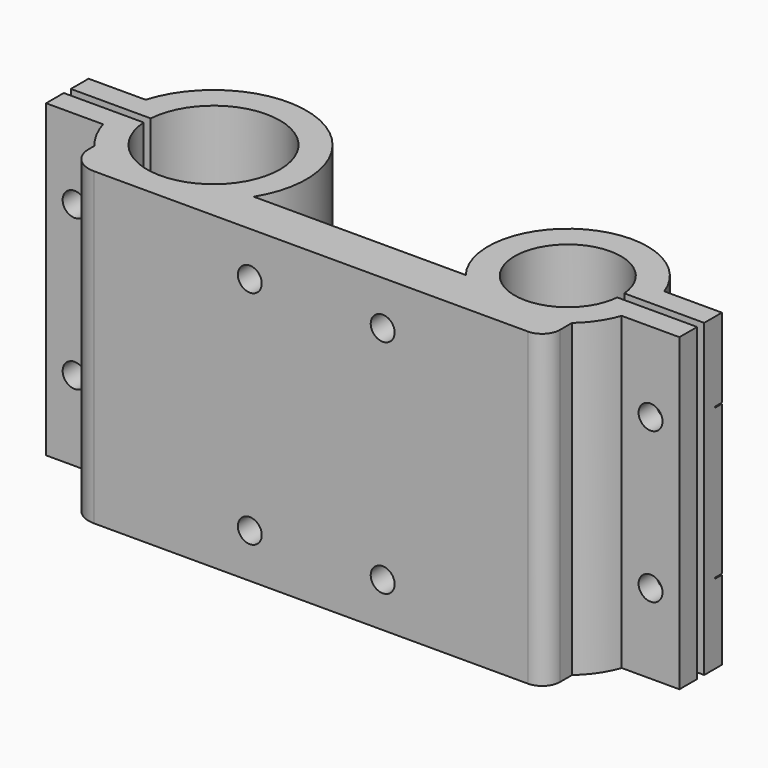
from build123d import *

# Parameters (mm, degrees)
F1_DEPTH   = 35
F3_D       = 2.7
F5_DEPTH   = 1
F6_DEPTH   = 1
F9_D       = 2.7
F9_ON_F7_D = 2.7
F8_W       = 1.6217698948
F8_H       = 2.85
F10_DEPTH  = 1
F11_DEPTH  = 1


# Not quite as in the source:
# - a feature names something its author has since deleted; it is built from what else it names


with BuildPart() as f1:
    # F0 (on Top) → F1 (new body)
    with BuildSketch(Plane.XY):
        with BuildLine():
            Line((-21.3074208284, -25.7097307226), (-27.8221394541, -25.7097307226))
            ThreePointArc((-27.8221394541, -25.7097307226), (-41.1900200037, -21.1492925546), (-42.5323706273, -35.2097307226))
            Line((-42.5323706273, -35.2097307226), (-68.0612095771, -35.2097307226))
            ThreePointArc((-68.0612095771, -35.2097307226), (-71.4714049121, -19.3897012131), (-86.3697267271, -25.7097307226))
            Line((-86.3697267271, -25.7097307226), (-92.8074208284, -25.7097307226))
            Line((-92.8074208284, -25.7097307226), (-92.8074208284, -28.2097307226))
            Line((-92.8074208284, -28.2097307226), (-83.7907356019, -28.2097307226))
            ThreePointArc((-83.7907356019, -28.2097307226), (-68.8074208284, -28.7097307226), (-83.7907356019, -29.2097307226))
            Line((-83.7907356019, -29.2097307226), (-92.8074208284, -29.2097307226))
            Line((-92.8074208284, -29.2097307226), (-92.8074208284, -31.7097307226))
            Line((-92.8074208284, -31.7097307226), (-86.3697267271, -31.7097307226))
            ThreePointArc((-86.3697267271, -31.7097307226), (-85.5676654464, -33.6592629847), (-84.3923404334, -35.4092885424))
            Line((-84.3923404334, -35.4092885424), (-84.3923404334, -36.2097307226))
            ThreePointArc((-84.3923404334, -36.2097307226), (-83.5136607769, -38.3310510662), (-81.3923404334, -39.2097307226))
            Line((-81.3923404334, -39.2097307226), (-32.3990289542, -39.2097307226))
            ThreePointArc((-32.3990289542, -39.2097307226), (-30.9848153918, -38.623944285), (-30.3990289542, -37.2097307226))
            Line((-30.3990289542, -37.2097307226), (-30.3990289542, -35.4987590376))
            ThreePointArc((-30.3990289542, -35.4987590376), (-28.8654021984, -33.7709913079), (-27.8221394541, -31.7097307226))
            Line((-27.8221394541, -31.7097307226), (-21.3074208284, -31.7097307226))
            Line((-21.3074208284, -31.7097307226), (-21.3074208284, -29.2097307226))
            Line((-21.3074208284, -29.2097307226), (-30.3282904568, -29.2097307226))
            ThreePointArc((-30.3282904568, -29.2097307226), (-42.3074208284, -28.7097307226), (-30.3282904568, -28.2097307226))
            Line((-30.3282904568, -28.2097307226), (-21.3074208284, -28.2097307226))
            Line((-21.3074208284, -28.2097307226), (-21.3074208284, -25.7097307226))
        make_face()
    extrude(amount=F1_DEPTH)

    # F3 (through all)
    with Locations(Plane.XZ.offset(39.2097307226)):
        with Locations((-63.8074208284, 30), (-48.80741708, 30), (-48.80741708, 5), (-63.8074208284, 5)):
            Hole(F3_D / 2)

    # F4 (on face) → F5 (cut)
    with BuildSketch(Plane(origin=(0, -35.2097307226, 0), x_dir=(-1, 0, 0), z_dir=(0, 1, 0))):
        Polygon((50.4817328606, 27.1), (52.1560486413, 30), (50.4817328606, 32.9), (47.1331012993, 32.9), (45.4587855187, 30), (47.1331012993, 27.1), align=None)
        Polygon((62.1331050477, 32.9), (60.4587892671, 30), (62.1331050477, 27.1), (65.481736609, 27.1), (67.1560523897, 30), (65.481736609, 32.9), align=None)
        Polygon((52.1560486413, 5), (50.4817328606, 7.9), (47.1331012993, 7.9), (45.4587855187, 5), (47.1331012993, 2.1), (50.4817328606, 2.1), align=None)
        Polygon((62.1331050477, 2.1), (65.481736609, 2.1), (67.1560523897, 5), (65.481736609, 7.9), (62.1331050477, 7.9), (60.4587892671, 5), align=None)
    extrude(amount=-F5_DEPTH, mode=Mode.SUBTRACT)

    # F6 (add): a face of the model
    f6_faces = [f1.faces().sort_by_distance(p)[0] for p in [
        (-55.1452142049, -35.2097307226, 17.5),
    ]]
    extrude(f6_faces, amount=F6_DEPTH)

    # F9 (through all)
    with Locations(Plane(origin=(0, -25.7097307226, 0), x_dir=(-1, 0, 0), z_dir=(0, 1, 0))):
        with Locations((24.5647801412, 26), (24.5647801412, 9)):
            Hole(F9_D / 2)

    # F9 on F7 (through all)
    with Locations(Plane(origin=(0, -25.7097307226, 0), x_dir=(-1, 0, 0), z_dir=(0, 1, 0))):
        with Locations((89.5885737777, 9), (89.5885737777, 26)):
            Hole(F9_ON_F7_D / 2)

    # F8 (on face) → F10 (cut)
    with BuildSketch(Plane(origin=(0, -25.7097307226, 0), x_dir=(-1, 0, 0), z_dir=(0, 1, 0))):
        Polygon((26.2102284084, 28.85), (24.5647801412, 28.85), (24.5647801412, 26), (26.1865500361, 26), (26.1865500361, 23.15), (26.2102284084, 23.15), (27.8556766756, 26), align=None)
        Polygon((24.5647801412, 26), (24.5647801412, 28.85), (22.919331874, 28.85), (21.2738836069, 26), (22.919331874, 23.15), (24.5647801412, 23.15), align=None)
        with Locations((25.3756650887, 10.425)):
            Rectangle(F8_W, F8_H)
        Polygon((24.5647801412, 9), (24.5647801412, 11.85), (22.919331874, 11.85), (21.2738836069, 9), (22.919331874, 6.15), (24.5647801412, 6.15), align=None)
        with Locations((25.3756650887, 24.575)):
            Rectangle(F8_W, F8_H)
        Polygon((26.1865500361, 9), (24.5647801412, 9), (24.5647801412, 6.15), (26.2102284084, 6.15), (27.8556766756, 9), (26.2102284084, 11.85), (26.1865500361, 11.85), align=None)
    extrude(amount=-F10_DEPTH, mode=Mode.SUBTRACT)

    # F7 (on face) → F11 (cut)
    with BuildSketch(Plane(origin=(0, -25.7097307226, 0), x_dir=(-1, 0, 0), z_dir=(0, 1, 0))):
        Polygon((91.2340220449, 6.15), (92.8794703121, 9), (91.2340220449, 11.85), (87.9431255105, 11.85), (86.2976772433, 9), (87.9431255105, 6.15), align=None)
        Polygon((92.8794703121, 26), (91.2340220449, 28.85), (87.9431255105, 28.85), (86.2976772433, 26), (87.9431255105, 23.15), (91.2340220449, 23.15), align=None)
    extrude(amount=-F11_DEPTH, mode=Mode.SUBTRACT)


solid = f1.part
